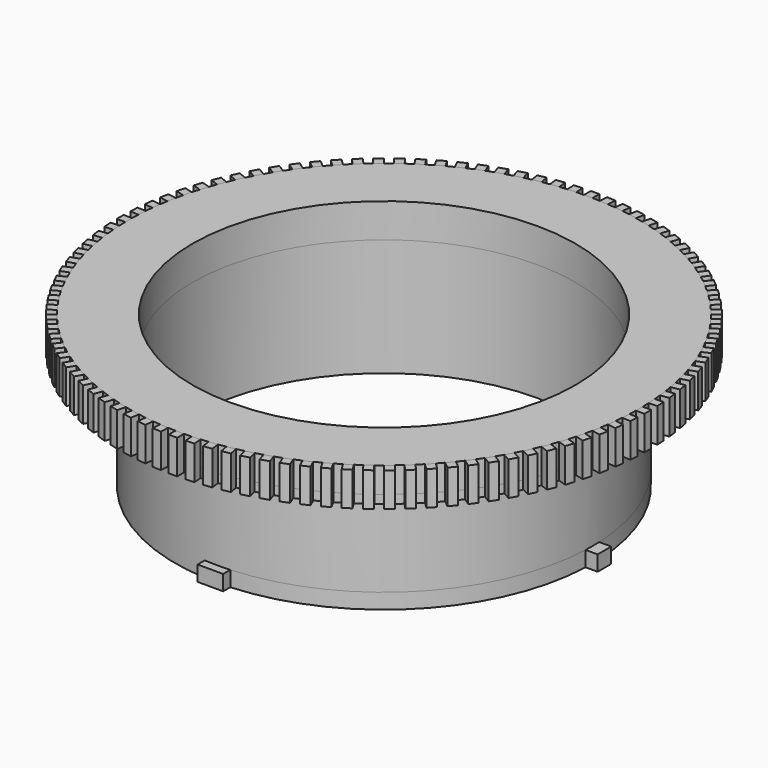
from build123d import *
from build123d import SkipClean  # not in build123d's __all__

# Parameters (mm, degrees)
F0_R     = 28.575
F1_DEPTH = 2.286
F2_R     = 31.115
F2_R_2   = 28.575
F3_DEPTH = 16.51
F4_R     = 38.1
F4_R_2   = 28.575
F5_DEPTH = 3.81
F6_R     = 28.575
F7_DEPTH = 5.08


with BuildPart() as f1:
    # F0 (on Top) → F1 (new body)
    with BuildSketch(Plane.XY):
        with BuildLine():
            Line((-2.54, 33.401), (-2.54, 31.0111532356))
            ThreePointArc((-2.54, 31.0111532356), (-31.1133717514, -0.3183131469), (-1.905, -31.056628922))
            Line((-1.905, -31.056628922), (-1.905, -32.385))
            Line((-1.905, -32.385), (1.905, -32.385))
            Line((1.905, -32.385), (1.905, -31.056628922))
            ThreePointArc((1.905, -31.056628922), (22.2252782457, -21.7756798264), (31.0890708288, -1.27))
            Line((31.0890708288, -1.27), (32.893, -1.27))
            Line((32.893, -1.27), (32.893, 1.27))
            Line((32.893, 1.27), (31.0890708288, 1.27))
            ThreePointArc((31.0890708288, 1.27), (22.4468850879, 21.5471709246), (2.54, 31.0111532356))
            Line((2.54, 31.0111532356), (2.54, 33.401))
            Line((2.54, 33.401), (-2.54, 33.401))
        make_face()
        Circle(F0_R, mode=Mode.SUBTRACT)
    extrude(amount=F1_DEPTH)

    # F2 (on face) → F3 (join)
    with BuildSketch(Plane.XY.offset(2.286)):
        Circle(F2_R)
        Circle(F2_R_2, mode=Mode.SUBTRACT)
    extrude(amount=F3_DEPTH)

    # F4 (on face) → F5 (join)
    with BuildSketch(Plane.XY.offset(18.796)):
        Circle(F4_R)
        Circle(F4_R_2, mode=Mode.SUBTRACT)
    extrude(amount=F5_DEPTH)

    # F6 (on face) → F7 (join)
    with BuildSketch(Plane.XY.offset(22.606)):
        with BuildLine():
            Line((0.635, -39.37), (0.635, -38.0947079658))
            ThreePointArc((0.635, -38.0947079658), (0, -38.1), (-0.635, -38.0947079658))
            Line((-0.635, -38.0947079658), (-0.635, -39.37))
            Line((-0.635, -39.37), (0.635, -39.37))
        make_face()
        with BuildLine():
            Line((3.1058097264, -39.2524403183), (3.025733477, -37.9796647816))
            ThreePointArc((3.025733477, -37.9796647816), (2.3923187941, -38.0248183531), (1.7582395319, -38.0594087414))
            Line((1.7582395319, -38.0594087414), (1.8383157813, -39.3321842781))
            Line((1.8383157813, -39.3321842781), (3.1058097264, -39.2524403183))
        make_face()
        with BuildLine():
            Line((5.5643622408, -38.9799691874), (5.4045257664, -37.7147332118))
            ThreePointArc((5.4045257664, -37.7147332118), (4.7751961988, -37.7995701201), (4.1445400957, -37.8739064185))
            Line((4.1445400957, -37.8739064185), (4.3043765701, -39.1391423941))
            Line((4.3043765701, -39.1391423941), (5.5643622408, -38.9799691874))
        make_face()
        with BuildLine():
            Line((8.0009547595, -38.5536619264), (7.7619888616, -37.3009588203))
            ThreePointArc((7.7619888616, -37.3009588203), (7.1392280857, -37.4251442528), (6.5144840532, -37.5389330898))
            Line((6.5144840532, -37.5389330898), (6.753449951, -38.791636196))
            Line((6.753449951, -38.791636196), (8.0009547595, -38.5536619264))
        make_face()
        with BuildLine():
            Line((10.405971165, -37.9752009753), (10.0888189329, -36.7399745854))
            ThreePointArc((10.0888189329, -36.7399745854), (9.475084701, -36.903018439), (8.8587183183, -37.0558107421))
            Line((8.8587183183, -37.0558107421), (9.1758705504, -38.291037132))
            Line((9.1758705504, -38.291037132), (10.405971165, -37.9752009753))
        make_face()
        with BuildLine():
            Line((12.7699199564, -37.2468692551), (12.375833045, -36.0339944558))
            ThreePointArc((12.375833045, -36.0339944558), (11.7735474857, -36.2352532708), (11.1679912693, -36.4264460387))
            Line((11.1679912693, -36.4264460387), (11.5620781807, -37.639320838))
            Line((11.5620781807, -37.639320838), (12.7699199564, -37.2468692551))
        make_face()
        with BuildLine():
            Line((15.0834717077, -36.3715411585), (14.6140053981, -35.1858046124))
            ThreePointArc((14.6140053981, -35.1858046124), (14.0255454573, -35.4244841123), (13.433189261, -35.6533227943))
            Line((13.433189261, -35.6533227943), (13.9026555707, -36.8390593404))
            Line((13.9026555707, -36.8390593404), (15.0834717077, -36.3715411585))
        make_face()
        with BuildLine():
            Line((17.3374958872, -35.3526712054), (16.7945029484, -34.1987524731))
            ThreePointArc((16.7945029484, -34.1987524731), (16.2221910086, -34.473910699), (15.6453725917, -34.7394921734))
            Line((15.6453725917, -34.7394921734), (16.1883655306, -35.8934109057))
            Line((16.1883655306, -35.8934109057), (17.3374958872, -35.3526712054))
        make_face()
        with BuildLine():
            Line((19.5230968912, -34.1942804103), (18.9087202682, -33.0767334817))
            ThreePointArc((18.9087202682, -33.0767334817), (18.3548149833, -33.3872845097), (17.7958107845, -33.6885606478))
            Line((17.7958107845, -33.6885606478), (18.4101874076, -34.8061075764))
            Line((18.4101874076, -34.8061075764), (19.5230968912, -34.1942804103))
        make_face()
        with BuildLine():
            Line((21.631649151, -32.9009404122), (20.9483135077, -31.8241757346))
            ThreePointArc((20.9483135077, -31.8241757346), (20.4150008887, -32.1688939616), (19.8760170423, -32.5046757642))
            Line((19.8760170423, -32.5046757642), (20.5593526856, -33.5814404418))
            Line((20.5593526856, -33.5814404418), (21.631649151, -32.9009404122))
        make_face()
        with BuildLine():
            Line((23.6548311742, -31.4777554333), (22.9052333241, -30.4460225049))
            ThreePointArc((22.9052333241, -30.4460225049), (22.3946181123, -30.8235474857), (21.8777817413, -31.1925097753))
            Line((21.8777817413, -31.1925097753), (22.6273795913, -32.2242427037))
            Line((22.6273795913, -32.2242427037), (23.6548311742, -31.4777554333))
        make_face()
        with BuildLine():
            Line((25.5846583856, -29.9303421346), (24.771756649, -28.9477127338))
            ThreePointArc((24.771756649, -28.9477127338), (24.2858540094, -29.3565545498), (23.7932048307, -29.7572412008))
            Line((23.7932048307, -29.7572412008), (24.6061065672, -30.7398706016))
            Line((24.6061065672, -30.7398706016), (25.5846583856, -29.9303421346))
        make_face()
        with BuildLine():
            Line((27.4135146388, -28.2648074493), (26.5405171676, -27.3351595656))
            ThreePointArc((26.5405171676, -27.3351595656), (26.0812447359, -27.7737047048), (25.6147270108, -28.2045343901))
            Line((25.6147270108, -28.2045343901), (26.487724482, -29.1341822738))
            Line((26.487724482, -29.1341822738), (27.4135146388, -28.2648074493))
        make_face()
        with BuildLine():
            Line((29.1341822738, -26.487724482), (28.2045343901, -25.6147270108))
            ThreePointArc((28.2045343901, -25.6147270108), (27.7737047048, -26.0812447359), (27.3351595656, -26.5405171676))
            Line((27.3351595656, -26.5405171676), (28.2648074493, -27.4135146388))
            Line((28.2648074493, -27.4135146388), (29.1341822738, -26.487724482))
        make_face()
        with BuildLine():
            Line((30.7398706016, -24.6061065672), (29.7572412008, -23.7932048307))
            ThreePointArc((29.7572412008, -23.7932048307), (29.3565545498, -24.2858540094), (28.9477127338, -24.771756649))
            Line((28.9477127338, -24.771756649), (29.9303421346, -25.5846583856))
            Line((29.9303421346, -25.5846583856), (30.7398706016, -24.6061065672))
        make_face()
        with BuildLine():
            Line((32.2242427037, -22.6273795913), (31.1925097753, -21.8777817413))
            ThreePointArc((31.1925097753, -21.8777817413), (30.8235474857, -22.3946181123), (30.4460225049, -22.9052333241))
            Line((30.4460225049, -22.9052333241), (31.4777554333, -23.6548311742))
            Line((31.4777554333, -23.6548311742), (32.2242427037, -22.6273795913))
        make_face()
        with BuildLine():
            Line((33.5814404418, -20.5593526856), (32.5046757642, -19.8760170423))
            ThreePointArc((32.5046757642, -19.8760170423), (32.1688939616, -20.4150008887), (31.8241757346, -20.9483135077))
            Line((31.8241757346, -20.9483135077), (32.9009404122, -21.631649151))
            Line((32.9009404122, -21.631649151), (33.5814404418, -20.5593526856))
        make_face()
        with BuildLine():
            Line((34.8061075764, -18.4101874076), (33.6885606478, -17.7958107845))
            ThreePointArc((33.6885606478, -17.7958107845), (33.3872845097, -18.3548149833), (33.0767334817, -18.9087202682))
            Line((33.0767334817, -18.9087202682), (34.1942804103, -19.5230968912))
            Line((34.1942804103, -19.5230968912), (34.8061075764, -18.4101874076))
        make_face()
        with BuildLine():
            Line((35.8934109057, -16.1883655306), (34.7394921734, -15.6453725917))
            ThreePointArc((34.7394921734, -15.6453725917), (34.473910699, -16.2221910086), (34.1987524731, -16.7945029484))
            Line((34.1987524731, -16.7945029484), (35.3526712054, -17.3374958872))
            Line((35.3526712054, -17.3374958872), (35.8934109057, -16.1883655306))
        make_face()
        with BuildLine():
            Line((36.8390593404, -13.9026555707), (35.6533227943, -13.433189261))
            ThreePointArc((35.6533227943, -13.433189261), (35.4244841123, -14.0255454573), (35.1858046124, -14.6140053981))
            Line((35.1858046124, -14.6140053981), (36.3715411585, -15.0834717077))
            Line((36.3715411585, -15.0834717077), (36.8390593404, -13.9026555707))
        make_face()
        with BuildLine():
            Line((37.639320838, -11.5620781807), (36.4264460387, -11.1679912693))
            ThreePointArc((36.4264460387, -11.1679912693), (36.2352532708, -11.7735474857), (36.0339944558, -12.375833045))
            Line((36.0339944558, -12.375833045), (37.2468692551, -12.7699199564))
            Line((37.2468692551, -12.7699199564), (37.639320838, -11.5620781807))
        make_face()
        with BuildLine():
            Line((38.291037132, -9.1758705504), (37.0558107421, -8.8587183183))
            ThreePointArc((37.0558107421, -8.8587183183), (36.903018439, -9.475084701), (36.7399745854, -10.0888189329))
            Line((36.7399745854, -10.0888189329), (37.9752009753, -10.405971165))
            Line((37.9752009753, -10.405971165), (38.291037132, -9.1758705504))
        make_face()
        with BuildLine():
            Line((38.791636196, -6.753449951), (37.5389330898, -6.5144840532))
            ThreePointArc((37.5389330898, -6.5144840532), (37.4251442528, -7.1392280857), (37.3009588203, -7.7619888616))
            Line((37.3009588203, -7.7619888616), (38.5536619264, -8.0009547595))
            Line((38.5536619264, -8.0009547595), (38.791636196, -6.753449951))
        make_face()
        with BuildLine():
            Line((39.1391423941, -4.3043765701), (37.8739064185, -4.1445400957))
            ThreePointArc((37.8739064185, -4.1445400957), (37.7995701201, -4.7751961988), (37.7147332118, -5.4045257664))
            Line((37.7147332118, -5.4045257664), (38.9799691874, -5.5643622408))
            Line((38.9799691874, -5.5643622408), (39.1391423941, -4.3043765701))
        make_face()
        with BuildLine():
            Line((39.3321842781, -1.8383157813), (38.0594087414, -1.7582395319))
            ThreePointArc((38.0594087414, -1.7582395319), (38.0248183531, -2.3923187941), (37.9796647816, -3.025733477))
            Line((37.9796647816, -3.025733477), (39.2524403183, -3.1058097264))
            Line((39.2524403183, -3.1058097264), (39.3321842781, -1.8383157813))
        make_face()
        with BuildLine():
            ThreePointArc((38.0947079658, 0.635), (38.0986769685, 0.3175110256), (38.1, 0))
            ThreePointArc((38.1, 0), (38.0986769685, -0.3175110256), (38.0947079658, -0.635))
            Line((38.0947079658, -0.635), (39.37, -0.635))
            Line((39.37, -0.635), (39.37, 0.635))
            Line((39.37, 0.635), (38.0947079658, 0.635))
        make_face()
        with BuildLine():
            ThreePointArc((37.9796647816, 3.025733477), (38.0248183531, 2.3923187941), (38.0594087414, 1.7582395319))
            Line((38.0594087414, 1.7582395319), (39.3321842781, 1.8383157813))
            Line((39.3321842781, 1.8383157813), (39.2524403183, 3.1058097264))
            Line((39.2524403183, 3.1058097264), (37.9796647816, 3.025733477))
        make_face()
        with BuildLine():
            ThreePointArc((37.7147332118, 5.4045257664), (37.7995701201, 4.7751961988), (37.8739064185, 4.1445400957))
            Line((37.8739064185, 4.1445400957), (39.1391423941, 4.3043765701))
            Line((39.1391423941, 4.3043765701), (38.9799691874, 5.5643622408))
            Line((38.9799691874, 5.5643622408), (37.7147332118, 5.4045257664))
        make_face()
        with BuildLine():
            ThreePointArc((37.3009588203, 7.7619888616), (37.4251442528, 7.1392280857), (37.5389330898, 6.5144840532))
            Line((37.5389330898, 6.5144840532), (38.791636196, 6.753449951))
            Line((38.791636196, 6.753449951), (38.5536619264, 8.0009547595))
            Line((38.5536619264, 8.0009547595), (37.3009588203, 7.7619888616))
        make_face()
        with BuildLine():
            ThreePointArc((36.7399745854, 10.0888189329), (36.903018439, 9.475084701), (37.0558107421, 8.8587183183))
            Line((37.0558107421, 8.8587183183), (38.291037132, 9.1758705504))
            Line((38.291037132, 9.1758705504), (37.9752009753, 10.405971165))
            Line((37.9752009753, 10.405971165), (36.7399745854, 10.0888189329))
        make_face()
        with BuildLine():
            ThreePointArc((36.0339944558, 12.375833045), (36.2352532708, 11.7735474857), (36.4264460387, 11.1679912693))
            Line((36.4264460387, 11.1679912693), (37.639320838, 11.5620781807))
            Line((37.639320838, 11.5620781807), (37.2468692551, 12.7699199564))
            Line((37.2468692551, 12.7699199564), (36.0339944558, 12.375833045))
        make_face()
        with BuildLine():
            ThreePointArc((35.1858046124, 14.6140053981), (35.4244841123, 14.0255454573), (35.6533227943, 13.433189261))
            Line((35.6533227943, 13.433189261), (36.8390593404, 13.9026555707))
            Line((36.8390593404, 13.9026555707), (36.3715411585, 15.0834717077))
            Line((36.3715411585, 15.0834717077), (35.1858046124, 14.6140053981))
        make_face()
        with BuildLine():
            ThreePointArc((34.1987524731, 16.7945029484), (34.473910699, 16.2221910086), (34.7394921734, 15.6453725917))
            Line((34.7394921734, 15.6453725917), (35.8934109057, 16.1883655306))
            Line((35.8934109057, 16.1883655306), (35.3526712054, 17.3374958872))
            Line((35.3526712054, 17.3374958872), (34.1987524731, 16.7945029484))
        make_face()
        with BuildLine():
            ThreePointArc((33.0767334817, 18.9087202682), (33.3872845097, 18.3548149833), (33.6885606478, 17.7958107845))
            Line((33.6885606478, 17.7958107845), (34.8061075764, 18.4101874076))
            Line((34.8061075764, 18.4101874076), (34.1942804103, 19.5230968912))
            Line((34.1942804103, 19.5230968912), (33.0767334817, 18.9087202682))
        make_face()
        with BuildLine():
            ThreePointArc((31.8241757346, 20.9483135077), (32.1688939616, 20.4150008887), (32.5046757642, 19.8760170423))
            Line((32.5046757642, 19.8760170423), (33.5814404418, 20.5593526856))
            Line((33.5814404418, 20.5593526856), (32.9009404122, 21.631649151))
            Line((32.9009404122, 21.631649151), (31.8241757346, 20.9483135077))
        make_face()
        with BuildLine():
            ThreePointArc((30.4460225049, 22.9052333241), (30.8235474857, 22.3946181123), (31.1925097753, 21.8777817413))
            Line((31.1925097753, 21.8777817413), (32.2242427037, 22.6273795913))
            Line((32.2242427037, 22.6273795913), (31.4777554333, 23.6548311742))
            Line((31.4777554333, 23.6548311742), (30.4460225049, 22.9052333241))
        make_face()
        with BuildLine():
            ThreePointArc((28.9477127338, 24.771756649), (29.3565545498, 24.2858540094), (29.7572412008, 23.7932048307))
            Line((29.7572412008, 23.7932048307), (30.7398706016, 24.6061065672))
            Line((30.7398706016, 24.6061065672), (29.9303421346, 25.5846583856))
            Line((29.9303421346, 25.5846583856), (28.9477127338, 24.771756649))
        make_face()
        with BuildLine():
            ThreePointArc((27.3351595656, 26.5405171676), (27.7737047048, 26.0812447359), (28.2045343901, 25.6147270108))
            Line((28.2045343901, 25.6147270108), (29.1341822738, 26.487724482))
            Line((29.1341822738, 26.487724482), (28.2648074493, 27.4135146388))
            Line((28.2648074493, 27.4135146388), (27.3351595656, 26.5405171676))
        make_face()
        with BuildLine():
            ThreePointArc((25.6147270108, 28.2045343901), (26.0812447359, 27.7737047048), (26.5405171676, 27.3351595656))
            Line((26.5405171676, 27.3351595656), (27.4135146388, 28.2648074493))
            Line((27.4135146388, 28.2648074493), (26.487724482, 29.1341822738))
            Line((26.487724482, 29.1341822738), (25.6147270108, 28.2045343901))
        make_face()
        with BuildLine():
            ThreePointArc((23.7932048307, 29.7572412008), (24.2858540094, 29.3565545498), (24.771756649, 28.9477127338))
            Line((24.771756649, 28.9477127338), (25.5846583856, 29.9303421346))
            Line((25.5846583856, 29.9303421346), (24.6061065672, 30.7398706016))
            Line((24.6061065672, 30.7398706016), (23.7932048307, 29.7572412008))
        make_face()
        with BuildLine():
            ThreePointArc((21.8777817413, 31.1925097753), (22.3946181123, 30.8235474857), (22.9052333241, 30.4460225049))
            Line((22.9052333241, 30.4460225049), (23.6548311742, 31.4777554333))
            Line((23.6548311742, 31.4777554333), (22.6273795913, 32.2242427037))
            Line((22.6273795913, 32.2242427037), (21.8777817413, 31.1925097753))
        make_face()
        with BuildLine():
            ThreePointArc((19.8760170423, 32.5046757642), (20.4150008887, 32.1688939616), (20.9483135077, 31.8241757346))
            Line((20.9483135077, 31.8241757346), (21.631649151, 32.9009404122))
            Line((21.631649151, 32.9009404122), (20.5593526856, 33.5814404418))
            Line((20.5593526856, 33.5814404418), (19.8760170423, 32.5046757642))
        make_face()
        with BuildLine():
            ThreePointArc((17.7958107845, 33.6885606478), (18.3548149833, 33.3872845097), (18.9087202682, 33.0767334817))
            Line((18.9087202682, 33.0767334817), (19.5230968912, 34.1942804103))
            Line((19.5230968912, 34.1942804103), (18.4101874076, 34.8061075764))
            Line((18.4101874076, 34.8061075764), (17.7958107845, 33.6885606478))
        make_face()
        with BuildLine():
            ThreePointArc((15.6453725917, 34.7394921734), (16.2221910086, 34.473910699), (16.7945029484, 34.1987524731))
            Line((16.7945029484, 34.1987524731), (17.3374958872, 35.3526712054))
            Line((17.3374958872, 35.3526712054), (16.1883655306, 35.8934109057))
            Line((16.1883655306, 35.8934109057), (15.6453725917, 34.7394921734))
        make_face()
        with BuildLine():
            ThreePointArc((13.433189261, 35.6533227943), (14.0255454573, 35.4244841123), (14.6140053981, 35.1858046124))
            Line((14.6140053981, 35.1858046124), (15.0834717077, 36.3715411585))
            Line((15.0834717077, 36.3715411585), (13.9026555707, 36.8390593404))
            Line((13.9026555707, 36.8390593404), (13.433189261, 35.6533227943))
        make_face()
        with BuildLine():
            ThreePointArc((11.1679912693, 36.4264460387), (11.7735474857, 36.2352532708), (12.375833045, 36.0339944558))
            Line((12.375833045, 36.0339944558), (12.7699199564, 37.2468692551))
            Line((12.7699199564, 37.2468692551), (11.5620781807, 37.639320838))
            Line((11.5620781807, 37.639320838), (11.1679912693, 36.4264460387))
        make_face()
        with BuildLine():
            ThreePointArc((8.8587183183, 37.0558107421), (9.475084701, 36.903018439), (10.0888189329, 36.7399745854))
            Line((10.0888189329, 36.7399745854), (10.405971165, 37.9752009753))
            Line((10.405971165, 37.9752009753), (9.1758705504, 38.291037132))
            Line((9.1758705504, 38.291037132), (8.8587183183, 37.0558107421))
        make_face()
        with BuildLine():
            ThreePointArc((6.5144840532, 37.5389330898), (7.1392280857, 37.4251442528), (7.7619888616, 37.3009588203))
            Line((7.7619888616, 37.3009588203), (8.0009547595, 38.5536619264))
            Line((8.0009547595, 38.5536619264), (6.753449951, 38.791636196))
            Line((6.753449951, 38.791636196), (6.5144840532, 37.5389330898))
        make_face()
        with BuildLine():
            ThreePointArc((4.1445400957, 37.8739064185), (4.7751961988, 37.7995701201), (5.4045257664, 37.7147332118))
            Line((5.4045257664, 37.7147332118), (5.5643622408, 38.9799691874))
            Line((5.5643622408, 38.9799691874), (4.3043765701, 39.1391423941))
            Line((4.3043765701, 39.1391423941), (4.1445400957, 37.8739064185))
        make_face()
        with BuildLine():
            ThreePointArc((1.7582395319, 38.0594087414), (2.3923187941, 38.0248183531), (3.025733477, 37.9796647816))
            Line((3.025733477, 37.9796647816), (3.1058097264, 39.2524403183))
            Line((3.1058097264, 39.2524403183), (1.8383157813, 39.3321842781))
            Line((1.8383157813, 39.3321842781), (1.7582395319, 38.0594087414))
        make_face()
        with BuildLine():
            ThreePointArc((-0.635, 38.0947079658), (0, 38.1), (0.635, 38.0947079658))
            Line((0.635, 38.0947079658), (0.635, 39.37))
            Line((0.635, 39.37), (-0.635, 39.37))
            Line((-0.635, 39.37), (-0.635, 38.0947079658))
        make_face()
        with BuildLine():
            ThreePointArc((-3.025733477, 37.9796647816), (-2.3923187941, 38.0248183531), (-1.7582395319, 38.0594087414))
            Line((-1.7582395319, 38.0594087414), (-1.8383157813, 39.3321842781))
            Line((-1.8383157813, 39.3321842781), (-3.1058097264, 39.2524403183))
            Line((-3.1058097264, 39.2524403183), (-3.025733477, 37.9796647816))
        make_face()
        with BuildLine():
            ThreePointArc((-5.4045257664, 37.7147332118), (-4.7751961988, 37.7995701201), (-4.1445400957, 37.8739064185))
            Line((-4.1445400957, 37.8739064185), (-4.3043765701, 39.1391423941))
            Line((-4.3043765701, 39.1391423941), (-5.5643622408, 38.9799691874))
            Line((-5.5643622408, 38.9799691874), (-5.4045257664, 37.7147332118))
        make_face()
        with BuildLine():
            ThreePointArc((-7.7619888616, 37.3009588203), (-7.1392280857, 37.4251442528), (-6.5144840532, 37.5389330898))
            Line((-6.5144840532, 37.5389330898), (-6.753449951, 38.791636196))
            Line((-6.753449951, 38.791636196), (-8.0009547595, 38.5536619264))
            Line((-8.0009547595, 38.5536619264), (-7.7619888616, 37.3009588203))
        make_face()
        with BuildLine():
            ThreePointArc((-10.0888189329, 36.7399745854), (-9.475084701, 36.903018439), (-8.8587183183, 37.0558107421))
            Line((-8.8587183183, 37.0558107421), (-9.1758705504, 38.291037132))
            Line((-9.1758705504, 38.291037132), (-10.405971165, 37.9752009753))
            Line((-10.405971165, 37.9752009753), (-10.0888189329, 36.7399745854))
        make_face()
        with BuildLine():
            ThreePointArc((-12.375833045, 36.0339944558), (-11.7735474857, 36.2352532708), (-11.1679912693, 36.4264460387))
            Line((-11.1679912693, 36.4264460387), (-11.5620781807, 37.639320838))
            Line((-11.5620781807, 37.639320838), (-12.7699199564, 37.2468692551))
            Line((-12.7699199564, 37.2468692551), (-12.375833045, 36.0339944558))
        make_face()
        with BuildLine():
            ThreePointArc((-14.6140053981, 35.1858046124), (-14.0255454573, 35.4244841123), (-13.433189261, 35.6533227943))
            Line((-13.433189261, 35.6533227943), (-13.9026555707, 36.8390593404))
            Line((-13.9026555707, 36.8390593404), (-15.0834717077, 36.3715411585))
            Line((-15.0834717077, 36.3715411585), (-14.6140053981, 35.1858046124))
        make_face()
        with BuildLine():
            ThreePointArc((-16.7945029484, 34.1987524731), (-16.2221910086, 34.473910699), (-15.6453725917, 34.7394921734))
            Line((-15.6453725917, 34.7394921734), (-16.1883655306, 35.8934109057))
            Line((-16.1883655306, 35.8934109057), (-17.3374958872, 35.3526712054))
            Line((-17.3374958872, 35.3526712054), (-16.7945029484, 34.1987524731))
        make_face()
        with BuildLine():
            ThreePointArc((-18.9087202682, 33.0767334817), (-18.3548149833, 33.3872845097), (-17.7958107845, 33.6885606478))
            Line((-17.7958107845, 33.6885606478), (-18.4101874076, 34.8061075764))
            Line((-18.4101874076, 34.8061075764), (-19.5230968912, 34.1942804103))
            Line((-19.5230968912, 34.1942804103), (-18.9087202682, 33.0767334817))
        make_face()
        with BuildLine():
            ThreePointArc((-20.9483135077, 31.8241757346), (-20.4150008887, 32.1688939616), (-19.8760170423, 32.5046757642))
            Line((-19.8760170423, 32.5046757642), (-20.5593526856, 33.5814404418))
            Line((-20.5593526856, 33.5814404418), (-21.631649151, 32.9009404122))
            Line((-21.631649151, 32.9009404122), (-20.9483135077, 31.8241757346))
        make_face()
        with BuildLine():
            ThreePointArc((-22.9052333241, 30.4460225049), (-22.3946181123, 30.8235474857), (-21.8777817413, 31.1925097753))
            Line((-21.8777817413, 31.1925097753), (-22.6273795913, 32.2242427037))
            Line((-22.6273795913, 32.2242427037), (-23.6548311742, 31.4777554333))
            Line((-23.6548311742, 31.4777554333), (-22.9052333241, 30.4460225049))
        make_face()
        with BuildLine():
            ThreePointArc((-24.771756649, 28.9477127338), (-24.2858540094, 29.3565545498), (-23.7932048307, 29.7572412008))
            Line((-23.7932048307, 29.7572412008), (-24.6061065672, 30.7398706016))
            Line((-24.6061065672, 30.7398706016), (-25.5846583856, 29.9303421346))
            Line((-25.5846583856, 29.9303421346), (-24.771756649, 28.9477127338))
        make_face()
        with BuildLine():
            ThreePointArc((-26.5405171676, 27.3351595656), (-26.0812447359, 27.7737047048), (-25.6147270108, 28.2045343901))
            Line((-25.6147270108, 28.2045343901), (-26.487724482, 29.1341822738))
            Line((-26.487724482, 29.1341822738), (-27.4135146388, 28.2648074493))
            Line((-27.4135146388, 28.2648074493), (-26.5405171676, 27.3351595656))
        make_face()
        with BuildLine():
            ThreePointArc((-28.2045343901, 25.6147270108), (-27.7737047048, 26.0812447359), (-27.3351595656, 26.5405171676))
            Line((-27.3351595656, 26.5405171676), (-28.2648074493, 27.4135146388))
            Line((-28.2648074493, 27.4135146388), (-29.1341822738, 26.487724482))
            Line((-29.1341822738, 26.487724482), (-28.2045343901, 25.6147270108))
        make_face()
        with BuildLine():
            ThreePointArc((-29.7572412008, 23.7932048307), (-29.3565545498, 24.2858540094), (-28.9477127338, 24.771756649))
            Line((-28.9477127338, 24.771756649), (-29.9303421346, 25.5846583856))
            Line((-29.9303421346, 25.5846583856), (-30.7398706016, 24.6061065672))
            Line((-30.7398706016, 24.6061065672), (-29.7572412008, 23.7932048307))
        make_face()
        with BuildLine():
            ThreePointArc((-31.1925097753, 21.8777817413), (-30.8235474857, 22.3946181123), (-30.4460225049, 22.9052333241))
            Line((-30.4460225049, 22.9052333241), (-31.4777554333, 23.6548311742))
            Line((-31.4777554333, 23.6548311742), (-32.2242427037, 22.6273795913))
            Line((-32.2242427037, 22.6273795913), (-31.1925097753, 21.8777817413))
        make_face()
        with BuildLine():
            ThreePointArc((-32.5046757642, 19.8760170423), (-32.1688939616, 20.4150008887), (-31.8241757346, 20.9483135077))
            Line((-31.8241757346, 20.9483135077), (-32.9009404122, 21.631649151))
            Line((-32.9009404122, 21.631649151), (-33.5814404418, 20.5593526856))
            Line((-33.5814404418, 20.5593526856), (-32.5046757642, 19.8760170423))
        make_face()
        with BuildLine():
            ThreePointArc((-33.6885606478, 17.7958107845), (-33.3872845097, 18.3548149833), (-33.0767334817, 18.9087202682))
            Line((-33.0767334817, 18.9087202682), (-34.1942804103, 19.5230968912))
            Line((-34.1942804103, 19.5230968912), (-34.8061075764, 18.4101874076))
            Line((-34.8061075764, 18.4101874076), (-33.6885606478, 17.7958107845))
        make_face()
        with BuildLine():
            ThreePointArc((-34.7394921734, 15.6453725917), (-34.473910699, 16.2221910086), (-34.1987524731, 16.7945029484))
            Line((-34.1987524731, 16.7945029484), (-35.3526712054, 17.3374958872))
            Line((-35.3526712054, 17.3374958872), (-35.8934109057, 16.1883655306))
            Line((-35.8934109057, 16.1883655306), (-34.7394921734, 15.6453725917))
        make_face()
        with BuildLine():
            ThreePointArc((-35.6533227943, 13.433189261), (-35.4244841123, 14.0255454573), (-35.1858046124, 14.6140053981))
            Line((-35.1858046124, 14.6140053981), (-36.3715411585, 15.0834717077))
            Line((-36.3715411585, 15.0834717077), (-36.8390593404, 13.9026555707))
            Line((-36.8390593404, 13.9026555707), (-35.6533227943, 13.433189261))
        make_face()
        with BuildLine():
            ThreePointArc((-36.4264460387, 11.1679912693), (-36.2352532708, 11.7735474857), (-36.0339944558, 12.375833045))
            Line((-36.0339944558, 12.375833045), (-37.2468692551, 12.7699199564))
            Line((-37.2468692551, 12.7699199564), (-37.639320838, 11.5620781807))
            Line((-37.639320838, 11.5620781807), (-36.4264460387, 11.1679912693))
        make_face()
        with BuildLine():
            ThreePointArc((-37.0558107421, 8.8587183183), (-36.903018439, 9.475084701), (-36.7399745854, 10.0888189329))
            Line((-36.7399745854, 10.0888189329), (-37.9752009753, 10.405971165))
            Line((-37.9752009753, 10.405971165), (-38.291037132, 9.1758705504))
            Line((-38.291037132, 9.1758705504), (-37.0558107421, 8.8587183183))
        make_face()
        with BuildLine():
            ThreePointArc((-37.5389330898, 6.5144840532), (-37.4251442528, 7.1392280857), (-37.3009588203, 7.7619888616))
            Line((-37.3009588203, 7.7619888616), (-38.5536619264, 8.0009547595))
            Line((-38.5536619264, 8.0009547595), (-38.791636196, 6.753449951))
            Line((-38.791636196, 6.753449951), (-37.5389330898, 6.5144840532))
        make_face()
        with BuildLine():
            ThreePointArc((-37.8739064185, 4.1445400957), (-37.7995701201, 4.7751961988), (-37.7147332118, 5.4045257664))
            Line((-37.7147332118, 5.4045257664), (-38.9799691874, 5.5643622408))
            Line((-38.9799691874, 5.5643622408), (-39.1391423941, 4.3043765701))
            Line((-39.1391423941, 4.3043765701), (-37.8739064185, 4.1445400957))
        make_face()
        with BuildLine():
            ThreePointArc((-38.0594087414, 1.7582395319), (-38.0248183531, 2.3923187941), (-37.9796647816, 3.025733477))
            Line((-37.9796647816, 3.025733477), (-39.2524403183, 3.1058097264))
            Line((-39.2524403183, 3.1058097264), (-39.3321842781, 1.8383157813))
            Line((-39.3321842781, 1.8383157813), (-38.0594087414, 1.7582395319))
        make_face()
        with BuildLine():
            ThreePointArc((-38.0947079658, -0.635), (-38.1, 0), (-38.0947079658, 0.635))
            Line((-38.0947079658, 0.635), (-39.37, 0.635))
            Line((-39.37, 0.635), (-39.37, -0.635))
            Line((-39.37, -0.635), (-38.0947079658, -0.635))
        make_face()
        with BuildLine():
            Line((-39.2524403183, -3.1058097264), (-37.9796647816, -3.025733477))
            ThreePointArc((-37.9796647816, -3.025733477), (-38.0248183531, -2.3923187941), (-38.0594087414, -1.7582395319))
            Line((-38.0594087414, -1.7582395319), (-39.3321842781, -1.8383157813))
            Line((-39.3321842781, -1.8383157813), (-39.2524403183, -3.1058097264))
        make_face()
        with BuildLine():
            Line((-38.9799691874, -5.5643622408), (-37.7147332118, -5.4045257664))
            ThreePointArc((-37.7147332118, -5.4045257664), (-37.7995701201, -4.7751961988), (-37.8739064185, -4.1445400957))
            Line((-37.8739064185, -4.1445400957), (-39.1391423941, -4.3043765701))
            Line((-39.1391423941, -4.3043765701), (-38.9799691874, -5.5643622408))
        make_face()
        with BuildLine():
            Line((-38.5536619264, -8.0009547595), (-37.3009588203, -7.7619888616))
            ThreePointArc((-37.3009588203, -7.7619888616), (-37.4251442528, -7.1392280857), (-37.5389330898, -6.5144840532))
            Line((-37.5389330898, -6.5144840532), (-38.791636196, -6.753449951))
            Line((-38.791636196, -6.753449951), (-38.5536619264, -8.0009547595))
        make_face()
        with BuildLine():
            Line((-37.9752009753, -10.405971165), (-36.7399745854, -10.0888189329))
            ThreePointArc((-36.7399745854, -10.0888189329), (-36.903018439, -9.475084701), (-37.0558107421, -8.8587183183))
            Line((-37.0558107421, -8.8587183183), (-38.291037132, -9.1758705504))
            Line((-38.291037132, -9.1758705504), (-37.9752009753, -10.405971165))
        make_face()
        with BuildLine():
            Line((-37.2468692551, -12.7699199564), (-36.0339944558, -12.375833045))
            ThreePointArc((-36.0339944558, -12.375833045), (-36.2352532708, -11.7735474857), (-36.4264460387, -11.1679912693))
            Line((-36.4264460387, -11.1679912693), (-37.639320838, -11.5620781807))
            Line((-37.639320838, -11.5620781807), (-37.2468692551, -12.7699199564))
        make_face()
        with BuildLine():
            Line((-36.3715411585, -15.0834717077), (-35.1858046124, -14.6140053981))
            ThreePointArc((-35.1858046124, -14.6140053981), (-35.4244841123, -14.0255454573), (-35.6533227943, -13.433189261))
            Line((-35.6533227943, -13.433189261), (-36.8390593404, -13.9026555707))
            Line((-36.8390593404, -13.9026555707), (-36.3715411585, -15.0834717077))
        make_face()
        with BuildLine():
            Line((-35.3526712054, -17.3374958872), (-34.1987524731, -16.7945029484))
            ThreePointArc((-34.1987524731, -16.7945029484), (-34.473910699, -16.2221910086), (-34.7394921734, -15.6453725917))
            Line((-34.7394921734, -15.6453725917), (-35.8934109057, -16.1883655306))
            Line((-35.8934109057, -16.1883655306), (-35.3526712054, -17.3374958872))
        make_face()
        with BuildLine():
            Line((-34.1942804103, -19.5230968912), (-33.0767334817, -18.9087202682))
            ThreePointArc((-33.0767334817, -18.9087202682), (-33.3872845097, -18.3548149833), (-33.6885606478, -17.7958107845))
            Line((-33.6885606478, -17.7958107845), (-34.8061075764, -18.4101874076))
            Line((-34.8061075764, -18.4101874076), (-34.1942804103, -19.5230968912))
        make_face()
        with BuildLine():
            Line((-32.9009404122, -21.631649151), (-31.8241757346, -20.9483135077))
            ThreePointArc((-31.8241757346, -20.9483135077), (-32.1688939616, -20.4150008887), (-32.5046757642, -19.8760170423))
            Line((-32.5046757642, -19.8760170423), (-33.5814404418, -20.5593526856))
            Line((-33.5814404418, -20.5593526856), (-32.9009404122, -21.631649151))
        make_face()
        with BuildLine():
            Line((-31.4777554333, -23.6548311742), (-30.4460225049, -22.9052333241))
            ThreePointArc((-30.4460225049, -22.9052333241), (-30.8235474857, -22.3946181123), (-31.1925097753, -21.8777817413))
            Line((-31.1925097753, -21.8777817413), (-32.2242427037, -22.6273795913))
            Line((-32.2242427037, -22.6273795913), (-31.4777554333, -23.6548311742))
        make_face()
        with BuildLine():
            Line((-29.9303421346, -25.5846583856), (-28.9477127338, -24.771756649))
            ThreePointArc((-28.9477127338, -24.771756649), (-29.3565545498, -24.2858540094), (-29.7572412008, -23.7932048307))
            Line((-29.7572412008, -23.7932048307), (-30.7398706016, -24.6061065672))
            Line((-30.7398706016, -24.6061065672), (-29.9303421346, -25.5846583856))
        make_face()
        with BuildLine():
            Line((-28.2648074493, -27.4135146388), (-27.3351595656, -26.5405171676))
            ThreePointArc((-27.3351595656, -26.5405171676), (-27.7737047048, -26.0812447359), (-28.2045343901, -25.6147270108))
            Line((-28.2045343901, -25.6147270108), (-29.1341822738, -26.487724482))
            Line((-29.1341822738, -26.487724482), (-28.2648074493, -27.4135146388))
        make_face()
        with BuildLine():
            Line((-26.487724482, -29.1341822738), (-25.6147270108, -28.2045343901))
            ThreePointArc((-25.6147270108, -28.2045343901), (-26.0812447359, -27.7737047048), (-26.5405171676, -27.3351595656))
            Line((-26.5405171676, -27.3351595656), (-27.4135146388, -28.2648074493))
            Line((-27.4135146388, -28.2648074493), (-26.487724482, -29.1341822738))
        make_face()
        with BuildLine():
            Line((-24.6061065672, -30.7398706016), (-23.7932048307, -29.7572412008))
            ThreePointArc((-23.7932048307, -29.7572412008), (-24.2858540094, -29.3565545498), (-24.771756649, -28.9477127338))
            Line((-24.771756649, -28.9477127338), (-25.5846583856, -29.9303421346))
            Line((-25.5846583856, -29.9303421346), (-24.6061065672, -30.7398706016))
        make_face()
        with BuildLine():
            Line((-22.6273795913, -32.2242427037), (-21.8777817413, -31.1925097753))
            ThreePointArc((-21.8777817413, -31.1925097753), (-22.3946181123, -30.8235474857), (-22.9052333241, -30.4460225049))
            Line((-22.9052333241, -30.4460225049), (-23.6548311742, -31.4777554333))
            Line((-23.6548311742, -31.4777554333), (-22.6273795913, -32.2242427037))
        make_face()
        with BuildLine():
            Line((-20.5593526856, -33.5814404418), (-19.8760170423, -32.5046757642))
            ThreePointArc((-19.8760170423, -32.5046757642), (-20.4150008887, -32.1688939616), (-20.9483135077, -31.8241757346))
            Line((-20.9483135077, -31.8241757346), (-21.631649151, -32.9009404122))
            Line((-21.631649151, -32.9009404122), (-20.5593526856, -33.5814404418))
        make_face()
        with BuildLine():
            Line((-18.4101874076, -34.8061075764), (-17.7958107845, -33.6885606478))
            ThreePointArc((-17.7958107845, -33.6885606478), (-18.3548149833, -33.3872845097), (-18.9087202682, -33.0767334817))
            Line((-18.9087202682, -33.0767334817), (-19.5230968912, -34.1942804103))
            Line((-19.5230968912, -34.1942804103), (-18.4101874076, -34.8061075764))
        make_face()
        with BuildLine():
            Line((-16.1883655306, -35.8934109057), (-15.6453725917, -34.7394921734))
            ThreePointArc((-15.6453725917, -34.7394921734), (-16.2221910086, -34.473910699), (-16.7945029484, -34.1987524731))
            Line((-16.7945029484, -34.1987524731), (-17.3374958872, -35.3526712054))
            Line((-17.3374958872, -35.3526712054), (-16.1883655306, -35.8934109057))
        make_face()
        with BuildLine():
            Line((-13.9026555707, -36.8390593404), (-13.433189261, -35.6533227943))
            ThreePointArc((-13.433189261, -35.6533227943), (-14.0255454573, -35.4244841123), (-14.6140053981, -35.1858046124))
            Line((-14.6140053981, -35.1858046124), (-15.0834717077, -36.3715411585))
            Line((-15.0834717077, -36.3715411585), (-13.9026555707, -36.8390593404))
        make_face()
        with BuildLine():
            Line((-11.5620781807, -37.639320838), (-11.1679912693, -36.4264460387))
            ThreePointArc((-11.1679912693, -36.4264460387), (-11.7735474857, -36.2352532708), (-12.375833045, -36.0339944558))
            Line((-12.375833045, -36.0339944558), (-12.7699199564, -37.2468692551))
            Line((-12.7699199564, -37.2468692551), (-11.5620781807, -37.639320838))
        make_face()
        with BuildLine():
            Line((-9.1758705504, -38.291037132), (-8.8587183183, -37.0558107421))
            ThreePointArc((-8.8587183183, -37.0558107421), (-9.475084701, -36.903018439), (-10.0888189329, -36.7399745854))
            Line((-10.0888189329, -36.7399745854), (-10.405971165, -37.9752009753))
            Line((-10.405971165, -37.9752009753), (-9.1758705504, -38.291037132))
        make_face()
        with BuildLine():
            Line((-6.753449951, -38.791636196), (-6.5144840532, -37.5389330898))
            ThreePointArc((-6.5144840532, -37.5389330898), (-7.1392280857, -37.4251442528), (-7.7619888616, -37.3009588203))
            Line((-7.7619888616, -37.3009588203), (-8.0009547595, -38.5536619264))
            Line((-8.0009547595, -38.5536619264), (-6.753449951, -38.791636196))
        make_face()
        with BuildLine():
            Line((-4.3043765701, -39.1391423941), (-4.1445400957, -37.8739064185))
            ThreePointArc((-4.1445400957, -37.8739064185), (-4.7751961988, -37.7995701201), (-5.4045257664, -37.7147332118))
            Line((-5.4045257664, -37.7147332118), (-5.5643622408, -38.9799691874))
            Line((-5.5643622408, -38.9799691874), (-4.3043765701, -39.1391423941))
        make_face()
        with BuildLine():
            Line((-1.8383157813, -39.3321842781), (-1.7582395319, -38.0594087414))
            ThreePointArc((-1.7582395319, -38.0594087414), (-2.3923187941, -38.0248183531), (-3.025733477, -37.9796647816))
            Line((-3.025733477, -37.9796647816), (-3.1058097264, -39.2524403183))
            Line((-3.1058097264, -39.2524403183), (-1.8383157813, -39.3321842781))
        make_face()
        with BuildLine():
            ThreePointArc((38.0947079658, -0.635), (38.0986769685, -0.3175110256), (38.1, 0))
            ThreePointArc((38.1, 0), (38.0986769685, 0.3175110256), (38.0947079658, 0.635))
            ThreePointArc((38.0947079658, 0.635), (38.0811999499, 1.1967499209), (38.0594087414, 1.7582395319))
            ThreePointArc((38.0594087414, 1.7582395319), (38.0248183531, 2.3923187941), (37.9796647816, 3.025733477))
            ThreePointArc((37.9796647816, 3.025733477), (37.9309108514, 3.5855267374), (37.8739064185, 4.1445400957))
            ThreePointArc((37.8739064185, 4.1445400957), (37.7995701201, 4.7751961988), (37.7147332118, 5.4045257664))
            ThreePointArc((37.7147332118, 5.4045257664), (37.6309257767, 5.960153118), (37.5389330898, 6.5144840532))
            ThreePointArc((37.5389330898, 6.5144840532), (37.4251442528, 7.1392280857), (37.3009588203, 7.7619888616))
            ThreePointArc((37.3009588203, 7.7619888616), (37.1824286299, 8.3112574972), (37.0558107421, 8.8587183183))
            ThreePointArc((37.0558107421, 8.8587183183), (36.903018439, 9.475084701), (36.7399745854, 10.0888189329))
            ThreePointArc((36.7399745854, 10.0888189329), (36.5871894243, 10.6295611401), (36.4264460387, 11.1679912693))
            ThreePointArc((36.4264460387, 11.1679912693), (36.2352532708, 11.7735474857), (36.0339944558, 12.375833045))
            ThreePointArc((36.0339944558, 12.375833045), (35.8475572972, 12.9059147613), (35.6533227943, 13.433189261))
            ThreePointArc((35.6533227943, 13.433189261), (35.4244841123, 14.0255454573), (35.1858046124, 14.6140053981))
            ThreePointArc((35.1858046124, 14.6140053981), (34.9664512386, 15.1313346332), (34.7394921734, 15.6453725917))
            ThreePointArc((34.7394921734, 15.6453725917), (34.473910699, 16.2221910086), (34.1987524731, 16.7945029484))
            ThreePointArc((34.1987524731, 16.7945029484), (33.9473485716, 17.2970380401), (33.6885606478, 17.7958107845))
            ThreePointArc((33.6885606478, 17.7958107845), (33.3872845097, 18.3548149833), (33.0767334817, 18.9087202682))
            ThreePointArc((33.0767334817, 18.9087202682), (32.7942712289, 19.3944779401), (32.5046757642, 19.8760170423))
            ThreePointArc((32.5046757642, 19.8760170423), (32.1688939616, 20.4150008887), (31.8241757346, 20.9483135077))
            ThreePointArc((31.8241757346, 20.9483135077), (31.5117698799, 21.4153766962), (31.1925097753, 21.8777817413))
            ThreePointArc((31.1925097753, 21.8777817413), (30.8235474857, 22.3946181123), (30.4460225049, 22.9052333241))
            ThreePointArc((30.4460225049, 22.9052333241), (30.1049059715, 23.3517587442), (29.7572412008, 23.7932048307))
            ThreePointArc((29.7572412008, 23.7932048307), (29.3565545498, 24.2858540094), (28.9477127338, 24.771756649))
            ThreePointArc((28.9477127338, 24.771756649), (28.5792317529, 25.1959820688), (28.2045343901, 25.6147270108))
            ThreePointArc((28.2045343901, 25.6147270108), (27.7737047048, 26.0812447359), (27.3351595656, 26.5405171676))
            ThreePointArc((27.3351595656, 26.5405171676), (26.9407683632, 26.9407683632), (26.5405171676, 27.3351595656))
            ThreePointArc((26.5405171676, 27.3351595656), (26.0812447359, 27.7737047048), (25.6147270108, 28.2045343901))
            ThreePointArc((25.6147270108, 28.2045343901), (25.1959820688, 28.5792317529), (24.771756649, 28.9477127338))
            ThreePointArc((24.771756649, 28.9477127338), (24.2858540094, 29.3565545498), (23.7932048307, 29.7572412008))
            ThreePointArc((23.7932048307, 29.7572412008), (23.3517587442, 30.1049059715), (22.9052333241, 30.4460225049))
            ThreePointArc((22.9052333241, 30.4460225049), (22.3946181123, 30.8235474857), (21.8777817413, 31.1925097753))
            ThreePointArc((21.8777817413, 31.1925097753), (21.4153766962, 31.5117698799), (20.9483135077, 31.8241757346))
            ThreePointArc((20.9483135077, 31.8241757346), (20.4150008887, 32.1688939616), (19.8760170423, 32.5046757642))
            ThreePointArc((19.8760170423, 32.5046757642), (19.3944779401, 32.7942712289), (18.9087202682, 33.0767334817))
            ThreePointArc((18.9087202682, 33.0767334817), (18.3548149833, 33.3872845097), (17.7958107845, 33.6885606478))
            ThreePointArc((17.7958107845, 33.6885606478), (17.2970380401, 33.9473485716), (16.7945029484, 34.1987524731))
            ThreePointArc((16.7945029484, 34.1987524731), (16.2221910086, 34.473910699), (15.6453725917, 34.7394921734))
            ThreePointArc((15.6453725917, 34.7394921734), (15.1313346332, 34.9664512386), (14.6140053981, 35.1858046124))
            ThreePointArc((14.6140053981, 35.1858046124), (14.0255454573, 35.4244841123), (13.433189261, 35.6533227943))
            ThreePointArc((13.433189261, 35.6533227943), (12.9059147613, 35.8475572972), (12.375833045, 36.0339944558))
            ThreePointArc((12.375833045, 36.0339944558), (11.7735474857, 36.2352532708), (11.1679912693, 36.4264460387))
            ThreePointArc((11.1679912693, 36.4264460387), (10.6295611401, 36.5871894243), (10.0888189329, 36.7399745854))
            ThreePointArc((10.0888189329, 36.7399745854), (9.475084701, 36.903018439), (8.8587183183, 37.0558107421))
            ThreePointArc((8.8587183183, 37.0558107421), (8.3112574972, 37.1824286299), (7.7619888616, 37.3009588203))
            ThreePointArc((7.7619888616, 37.3009588203), (7.1392280857, 37.4251442528), (6.5144840532, 37.5389330898))
            ThreePointArc((6.5144840532, 37.5389330898), (5.960153118, 37.6309257767), (5.4045257664, 37.7147332118))
            ThreePointArc((5.4045257664, 37.7147332118), (4.7751961988, 37.7995701201), (4.1445400957, 37.8739064185))
            ThreePointArc((4.1445400957, 37.8739064185), (3.5855267374, 37.9309108514), (3.025733477, 37.9796647816))
            ThreePointArc((3.025733477, 37.9796647816), (2.3923187941, 38.0248183531), (1.7582395319, 38.0594087414))
            ThreePointArc((1.7582395319, 38.0594087414), (1.1967499209, 38.0811999499), (0.635, 38.0947079658))
            ThreePointArc((0.635, 38.0947079658), (0, 38.1), (-0.635, 38.0947079658))
            ThreePointArc((-0.635, 38.0947079658), (-1.1967499209, 38.0811999499), (-1.7582395319, 38.0594087414))
            ThreePointArc((-1.7582395319, 38.0594087414), (-2.3923187941, 38.0248183531), (-3.025733477, 37.9796647816))
            ThreePointArc((-3.025733477, 37.9796647816), (-3.5855267374, 37.9309108514), (-4.1445400957, 37.8739064185))
            ThreePointArc((-4.1445400957, 37.8739064185), (-4.7751961988, 37.7995701201), (-5.4045257664, 37.7147332118))
            ThreePointArc((-5.4045257664, 37.7147332118), (-5.960153118, 37.6309257767), (-6.5144840532, 37.5389330898))
            ThreePointArc((-6.5144840532, 37.5389330898), (-7.1392280857, 37.4251442528), (-7.7619888616, 37.3009588203))
            ThreePointArc((-7.7619888616, 37.3009588203), (-8.3112574972, 37.1824286299), (-8.8587183183, 37.0558107421))
            ThreePointArc((-8.8587183183, 37.0558107421), (-9.475084701, 36.903018439), (-10.0888189329, 36.7399745854))
            ThreePointArc((-10.0888189329, 36.7399745854), (-10.6295611401, 36.5871894243), (-11.1679912693, 36.4264460387))
            ThreePointArc((-11.1679912693, 36.4264460387), (-11.7735474857, 36.2352532708), (-12.375833045, 36.0339944558))
            ThreePointArc((-12.375833045, 36.0339944558), (-12.9059147613, 35.8475572972), (-13.433189261, 35.6533227943))
            ThreePointArc((-13.433189261, 35.6533227943), (-14.0255454573, 35.4244841123), (-14.6140053981, 35.1858046124))
            ThreePointArc((-14.6140053981, 35.1858046124), (-15.1313346332, 34.9664512386), (-15.6453725917, 34.7394921734))
            ThreePointArc((-15.6453725917, 34.7394921734), (-16.2221910086, 34.473910699), (-16.7945029484, 34.1987524731))
            ThreePointArc((-16.7945029484, 34.1987524731), (-17.2970380401, 33.9473485716), (-17.7958107845, 33.6885606478))
            ThreePointArc((-17.7958107845, 33.6885606478), (-18.3548149833, 33.3872845097), (-18.9087202682, 33.0767334817))
            ThreePointArc((-18.9087202682, 33.0767334817), (-19.3944779401, 32.7942712289), (-19.8760170423, 32.5046757642))
            ThreePointArc((-19.8760170423, 32.5046757642), (-20.4150008887, 32.1688939616), (-20.9483135077, 31.8241757346))
            ThreePointArc((-20.9483135077, 31.8241757346), (-21.4153766962, 31.5117698799), (-21.8777817413, 31.1925097753))
            ThreePointArc((-21.8777817413, 31.1925097753), (-22.3946181123, 30.8235474857), (-22.9052333241, 30.4460225049))
            ThreePointArc((-22.9052333241, 30.4460225049), (-23.3517587442, 30.1049059715), (-23.7932048307, 29.7572412008))
            ThreePointArc((-23.7932048307, 29.7572412008), (-24.2858540094, 29.3565545498), (-24.771756649, 28.9477127338))
            ThreePointArc((-24.771756649, 28.9477127338), (-25.1959820688, 28.5792317529), (-25.6147270108, 28.2045343901))
            ThreePointArc((-25.6147270108, 28.2045343901), (-26.0812447359, 27.7737047048), (-26.5405171676, 27.3351595656))
            ThreePointArc((-26.5405171676, 27.3351595656), (-26.9407683632, 26.9407683632), (-27.3351595656, 26.5405171676))
            ThreePointArc((-27.3351595656, 26.5405171676), (-27.7737047048, 26.0812447359), (-28.2045343901, 25.6147270108))
            ThreePointArc((-28.2045343901, 25.6147270108), (-28.5792317529, 25.1959820688), (-28.9477127338, 24.771756649))
            ThreePointArc((-28.9477127338, 24.771756649), (-29.3565545498, 24.2858540094), (-29.7572412008, 23.7932048307))
            ThreePointArc((-29.7572412008, 23.7932048307), (-30.1049059715, 23.3517587442), (-30.4460225049, 22.9052333241))
            ThreePointArc((-30.4460225049, 22.9052333241), (-30.8235474857, 22.3946181123), (-31.1925097753, 21.8777817413))
            ThreePointArc((-31.1925097753, 21.8777817413), (-31.5117698799, 21.4153766962), (-31.8241757346, 20.9483135077))
            ThreePointArc((-31.8241757346, 20.9483135077), (-32.1688939616, 20.4150008887), (-32.5046757642, 19.8760170423))
            ThreePointArc((-32.5046757642, 19.8760170423), (-32.7942712289, 19.3944779401), (-33.0767334817, 18.9087202682))
            ThreePointArc((-33.0767334817, 18.9087202682), (-33.3872845097, 18.3548149833), (-33.6885606478, 17.7958107845))
            ThreePointArc((-33.6885606478, 17.7958107845), (-33.9473485716, 17.2970380401), (-34.1987524731, 16.7945029484))
            ThreePointArc((-34.1987524731, 16.7945029484), (-34.473910699, 16.2221910086), (-34.7394921734, 15.6453725917))
            ThreePointArc((-34.7394921734, 15.6453725917), (-34.9664512386, 15.1313346332), (-35.1858046124, 14.6140053981))
            ThreePointArc((-35.1858046124, 14.6140053981), (-35.4244841123, 14.0255454573), (-35.6533227943, 13.433189261))
            ThreePointArc((-35.6533227943, 13.433189261), (-35.8475572972, 12.9059147613), (-36.0339944558, 12.375833045))
            ThreePointArc((-36.0339944558, 12.375833045), (-36.2352532708, 11.7735474857), (-36.4264460387, 11.1679912693))
            ThreePointArc((-36.4264460387, 11.1679912693), (-36.5871894243, 10.6295611401), (-36.7399745854, 10.0888189329))
            ThreePointArc((-36.7399745854, 10.0888189329), (-36.903018439, 9.475084701), (-37.0558107421, 8.8587183183))
            ThreePointArc((-37.0558107421, 8.8587183183), (-37.1824286299, 8.3112574972), (-37.3009588203, 7.7619888616))
            ThreePointArc((-37.3009588203, 7.7619888616), (-37.4251442528, 7.1392280857), (-37.5389330898, 6.5144840532))
            ThreePointArc((-37.5389330898, 6.5144840532), (-37.6309257767, 5.960153118), (-37.7147332118, 5.4045257664))
            ThreePointArc((-37.7147332118, 5.4045257664), (-37.7995701201, 4.7751961988), (-37.8739064185, 4.1445400957))
            ThreePointArc((-37.8739064185, 4.1445400957), (-37.9309108514, 3.5855267374), (-37.9796647816, 3.025733477))
            ThreePointArc((-37.9796647816, 3.025733477), (-38.0248183531, 2.3923187941), (-38.0594087414, 1.7582395319))
            ThreePointArc((-38.0594087414, 1.7582395319), (-38.0811999499, 1.1967499209), (-38.0947079658, 0.635))
            ThreePointArc((-38.0947079658, 0.635), (-38.1, 0), (-38.0947079658, -0.635))
            ThreePointArc((-38.0947079658, -0.635), (-38.0811999499, -1.1967499209), (-38.0594087414, -1.7582395319))
            ThreePointArc((-38.0594087414, -1.7582395319), (-38.0248183531, -2.3923187941), (-37.9796647816, -3.025733477))
            ThreePointArc((-37.9796647816, -3.025733477), (-37.9309108514, -3.5855267374), (-37.8739064185, -4.1445400957))
            ThreePointArc((-37.8739064185, -4.1445400957), (-37.7995701201, -4.7751961988), (-37.7147332118, -5.4045257664))
            ThreePointArc((-37.7147332118, -5.4045257664), (-37.6309257767, -5.960153118), (-37.5389330898, -6.5144840532))
            ThreePointArc((-37.5389330898, -6.5144840532), (-37.4251442528, -7.1392280857), (-37.3009588203, -7.7619888616))
            ThreePointArc((-37.3009588203, -7.7619888616), (-37.1824286299, -8.3112574972), (-37.0558107421, -8.8587183183))
            ThreePointArc((-37.0558107421, -8.8587183183), (-36.903018439, -9.475084701), (-36.7399745854, -10.0888189329))
            ThreePointArc((-36.7399745854, -10.0888189329), (-36.5871894243, -10.6295611401), (-36.4264460387, -11.1679912693))
            ThreePointArc((-36.4264460387, -11.1679912693), (-36.2352532708, -11.7735474857), (-36.0339944558, -12.375833045))
            ThreePointArc((-36.0339944558, -12.375833045), (-35.8475572972, -12.9059147613), (-35.6533227943, -13.433189261))
            ThreePointArc((-35.6533227943, -13.433189261), (-35.4244841123, -14.0255454573), (-35.1858046124, -14.6140053981))
            ThreePointArc((-35.1858046124, -14.6140053981), (-34.9664512386, -15.1313346332), (-34.7394921734, -15.6453725917))
            ThreePointArc((-34.7394921734, -15.6453725917), (-34.473910699, -16.2221910086), (-34.1987524731, -16.7945029484))
            ThreePointArc((-34.1987524731, -16.7945029484), (-33.9473485716, -17.2970380401), (-33.6885606478, -17.7958107845))
            ThreePointArc((-33.6885606478, -17.7958107845), (-33.3872845097, -18.3548149833), (-33.0767334817, -18.9087202682))
            ThreePointArc((-33.0767334817, -18.9087202682), (-32.7942712289, -19.3944779401), (-32.5046757642, -19.8760170423))
            ThreePointArc((-32.5046757642, -19.8760170423), (-32.1688939616, -20.4150008887), (-31.8241757346, -20.9483135077))
            ThreePointArc((-31.8241757346, -20.9483135077), (-31.5117698799, -21.4153766962), (-31.1925097753, -21.8777817413))
            ThreePointArc((-31.1925097753, -21.8777817413), (-30.8235474857, -22.3946181123), (-30.4460225049, -22.9052333241))
            ThreePointArc((-30.4460225049, -22.9052333241), (-30.1049059715, -23.3517587442), (-29.7572412008, -23.7932048307))
            ThreePointArc((-29.7572412008, -23.7932048307), (-29.3565545498, -24.2858540094), (-28.9477127338, -24.771756649))
            ThreePointArc((-28.9477127338, -24.771756649), (-28.5792317529, -25.1959820688), (-28.2045343901, -25.6147270108))
            ThreePointArc((-28.2045343901, -25.6147270108), (-27.7737047048, -26.0812447359), (-27.3351595656, -26.5405171676))
            ThreePointArc((-27.3351595656, -26.5405171676), (-26.9407683632, -26.9407683632), (-26.5405171676, -27.3351595656))
            ThreePointArc((-26.5405171676, -27.3351595656), (-26.0812447359, -27.7737047048), (-25.6147270108, -28.2045343901))
            ThreePointArc((-25.6147270108, -28.2045343901), (-25.1959820688, -28.5792317529), (-24.771756649, -28.9477127338))
            ThreePointArc((-24.771756649, -28.9477127338), (-24.2858540094, -29.3565545498), (-23.7932048307, -29.7572412008))
            ThreePointArc((-23.7932048307, -29.7572412008), (-23.3517587442, -30.1049059715), (-22.9052333241, -30.4460225049))
            ThreePointArc((-22.9052333241, -30.4460225049), (-22.3946181123, -30.8235474857), (-21.8777817413, -31.1925097753))
            ThreePointArc((-21.8777817413, -31.1925097753), (-21.4153766962, -31.5117698799), (-20.9483135077, -31.8241757346))
            ThreePointArc((-20.9483135077, -31.8241757346), (-20.4150008887, -32.1688939616), (-19.8760170423, -32.5046757642))
            ThreePointArc((-19.8760170423, -32.5046757642), (-19.3944779401, -32.7942712289), (-18.9087202682, -33.0767334817))
            ThreePointArc((-18.9087202682, -33.0767334817), (-18.3548149833, -33.3872845097), (-17.7958107845, -33.6885606478))
            ThreePointArc((-17.7958107845, -33.6885606478), (-17.2970380401, -33.9473485716), (-16.7945029484, -34.1987524731))
            ThreePointArc((-16.7945029484, -34.1987524731), (-16.2221910086, -34.473910699), (-15.6453725917, -34.7394921734))
            ThreePointArc((-15.6453725917, -34.7394921734), (-15.1313346332, -34.9664512386), (-14.6140053981, -35.1858046124))
            ThreePointArc((-14.6140053981, -35.1858046124), (-14.0255454573, -35.4244841123), (-13.433189261, -35.6533227943))
            ThreePointArc((-13.433189261, -35.6533227943), (-12.9059147613, -35.8475572972), (-12.375833045, -36.0339944558))
            ThreePointArc((-12.375833045, -36.0339944558), (-11.7735474857, -36.2352532708), (-11.1679912693, -36.4264460387))
            ThreePointArc((-11.1679912693, -36.4264460387), (-10.6295611401, -36.5871894243), (-10.0888189329, -36.7399745854))
            ThreePointArc((-10.0888189329, -36.7399745854), (-9.475084701, -36.903018439), (-8.8587183183, -37.0558107421))
            ThreePointArc((-8.8587183183, -37.0558107421), (-8.3112574972, -37.1824286299), (-7.7619888616, -37.3009588203))
            ThreePointArc((-7.7619888616, -37.3009588203), (-7.1392280857, -37.4251442528), (-6.5144840532, -37.5389330898))
            ThreePointArc((-6.5144840532, -37.5389330898), (-5.960153118, -37.6309257767), (-5.4045257664, -37.7147332118))
            ThreePointArc((-5.4045257664, -37.7147332118), (-4.7751961988, -37.7995701201), (-4.1445400957, -37.8739064185))
            ThreePointArc((-4.1445400957, -37.8739064185), (-3.5855267374, -37.9309108514), (-3.025733477, -37.9796647816))
            ThreePointArc((-3.025733477, -37.9796647816), (-2.3923187941, -38.0248183531), (-1.7582395319, -38.0594087414))
            ThreePointArc((-1.7582395319, -38.0594087414), (-1.1967499209, -38.0811999499), (-0.635, -38.0947079658))
            ThreePointArc((-0.635, -38.0947079658), (0, -38.1), (0.635, -38.0947079658))
            ThreePointArc((0.635, -38.0947079658), (1.1967499209, -38.0811999499), (1.7582395319, -38.0594087414))
            ThreePointArc((1.7582395319, -38.0594087414), (2.3923187941, -38.0248183531), (3.025733477, -37.9796647816))
            ThreePointArc((3.025733477, -37.9796647816), (3.5855267374, -37.9309108514), (4.1445400957, -37.8739064185))
            ThreePointArc((4.1445400957, -37.8739064185), (4.7751961988, -37.7995701201), (5.4045257664, -37.7147332118))
            ThreePointArc((5.4045257664, -37.7147332118), (5.960153118, -37.6309257767), (6.5144840532, -37.5389330898))
            ThreePointArc((6.5144840532, -37.5389330898), (7.1392280857, -37.4251442528), (7.7619888616, -37.3009588203))
            ThreePointArc((7.7619888616, -37.3009588203), (8.3112574972, -37.1824286299), (8.8587183183, -37.0558107421))
            ThreePointArc((8.8587183183, -37.0558107421), (9.475084701, -36.903018439), (10.0888189329, -36.7399745854))
            ThreePointArc((10.0888189329, -36.7399745854), (10.6295611401, -36.5871894243), (11.1679912693, -36.4264460387))
            ThreePointArc((11.1679912693, -36.4264460387), (11.7735474857, -36.2352532708), (12.375833045, -36.0339944558))
            ThreePointArc((12.375833045, -36.0339944558), (12.9059147613, -35.8475572972), (13.433189261, -35.6533227943))
            ThreePointArc((13.433189261, -35.6533227943), (14.0255454573, -35.4244841123), (14.6140053981, -35.1858046124))
            ThreePointArc((14.6140053981, -35.1858046124), (15.1313346332, -34.9664512386), (15.6453725917, -34.7394921734))
            ThreePointArc((15.6453725917, -34.7394921734), (16.2221910086, -34.473910699), (16.7945029484, -34.1987524731))
            ThreePointArc((16.7945029484, -34.1987524731), (17.2970380401, -33.9473485716), (17.7958107845, -33.6885606478))
            ThreePointArc((17.7958107845, -33.6885606478), (18.3548149833, -33.3872845097), (18.9087202682, -33.0767334817))
            ThreePointArc((18.9087202682, -33.0767334817), (19.3944779401, -32.7942712289), (19.8760170423, -32.5046757642))
            ThreePointArc((19.8760170423, -32.5046757642), (20.4150008887, -32.1688939616), (20.9483135077, -31.8241757346))
            ThreePointArc((20.9483135077, -31.8241757346), (21.4153766962, -31.5117698799), (21.8777817413, -31.1925097753))
            ThreePointArc((21.8777817413, -31.1925097753), (22.3946181123, -30.8235474857), (22.9052333241, -30.4460225049))
            ThreePointArc((22.9052333241, -30.4460225049), (23.3517587442, -30.1049059715), (23.7932048307, -29.7572412008))
            ThreePointArc((23.7932048307, -29.7572412008), (24.2858540094, -29.3565545498), (24.771756649, -28.9477127338))
            ThreePointArc((24.771756649, -28.9477127338), (25.1959820688, -28.5792317529), (25.6147270108, -28.2045343901))
            ThreePointArc((25.6147270108, -28.2045343901), (26.0812447359, -27.7737047048), (26.5405171676, -27.3351595656))
            ThreePointArc((26.5405171676, -27.3351595656), (26.9407683632, -26.9407683632), (27.3351595656, -26.5405171676))
            ThreePointArc((27.3351595656, -26.5405171676), (27.7737047048, -26.0812447359), (28.2045343901, -25.6147270108))
            ThreePointArc((28.2045343901, -25.6147270108), (28.5792317529, -25.1959820688), (28.9477127338, -24.771756649))
            ThreePointArc((28.9477127338, -24.771756649), (29.3565545498, -24.2858540094), (29.7572412008, -23.7932048307))
            ThreePointArc((29.7572412008, -23.7932048307), (30.1049059715, -23.3517587442), (30.4460225049, -22.9052333241))
            ThreePointArc((30.4460225049, -22.9052333241), (30.8235474857, -22.3946181123), (31.1925097753, -21.8777817413))
            ThreePointArc((31.1925097753, -21.8777817413), (31.5117698799, -21.4153766962), (31.8241757346, -20.9483135077))
            ThreePointArc((31.8241757346, -20.9483135077), (32.1688939616, -20.4150008887), (32.5046757642, -19.8760170423))
            ThreePointArc((32.5046757642, -19.8760170423), (32.7942712289, -19.3944779401), (33.0767334817, -18.9087202682))
            ThreePointArc((33.0767334817, -18.9087202682), (33.3872845097, -18.3548149833), (33.6885606478, -17.7958107845))
            ThreePointArc((33.6885606478, -17.7958107845), (33.9473485716, -17.2970380401), (34.1987524731, -16.7945029484))
            ThreePointArc((34.1987524731, -16.7945029484), (34.473910699, -16.2221910086), (34.7394921734, -15.6453725917))
            ThreePointArc((34.7394921734, -15.6453725917), (34.9664512386, -15.1313346332), (35.1858046124, -14.6140053981))
            ThreePointArc((35.1858046124, -14.6140053981), (35.4244841123, -14.0255454573), (35.6533227943, -13.433189261))
            ThreePointArc((35.6533227943, -13.433189261), (35.8475572972, -12.9059147613), (36.0339944558, -12.375833045))
            ThreePointArc((36.0339944558, -12.375833045), (36.2352532708, -11.7735474857), (36.4264460387, -11.1679912693))
            ThreePointArc((36.4264460387, -11.1679912693), (36.5871894243, -10.6295611401), (36.7399745854, -10.0888189329))
            ThreePointArc((36.7399745854, -10.0888189329), (36.903018439, -9.475084701), (37.0558107421, -8.8587183183))
            ThreePointArc((37.0558107421, -8.8587183183), (37.1824286299, -8.3112574972), (37.3009588203, -7.7619888616))
            ThreePointArc((37.3009588203, -7.7619888616), (37.4251442528, -7.1392280857), (37.5389330898, -6.5144840532))
            ThreePointArc((37.5389330898, -6.5144840532), (37.6309257767, -5.960153118), (37.7147332118, -5.4045257664))
            ThreePointArc((37.7147332118, -5.4045257664), (37.7995701201, -4.7751961988), (37.8739064185, -4.1445400957))
            ThreePointArc((37.8739064185, -4.1445400957), (37.9309108514, -3.5855267374), (37.9796647816, -3.025733477))
            ThreePointArc((37.9796647816, -3.025733477), (38.0248183531, -2.3923187941), (38.0594087414, -1.7582395319))
            ThreePointArc((38.0594087414, -1.7582395319), (38.0811999499, -1.1967499209), (38.0947079658, -0.635))
        make_face()
        Circle(F6_R, mode=Mode.SUBTRACT)
    with SkipClean():  # cleaning this boolean's faces spoils the solid; the shape is the same uncleaned
        extrude(amount=-F7_DEPTH)


solid = f1.part
